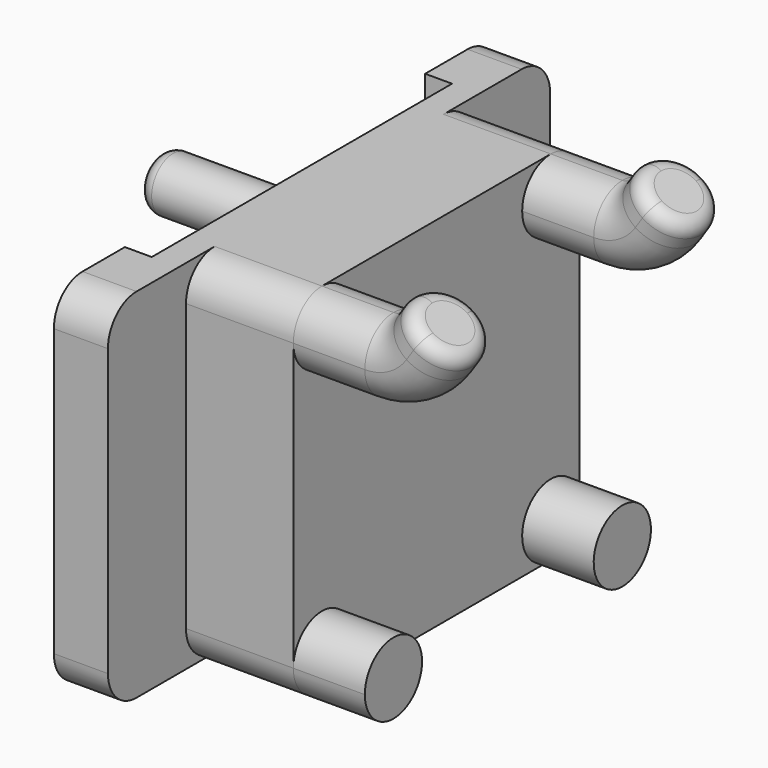
from build123d import *

# Parameters (mm, degrees)
F0_W      = 31.75
F0_H      = 31.75
F1_DEPTH  = 9.525
F7_R      = 1.27
F11_DEPTH = 6.35
F12_R     = 3.1749
F14_DEPTH = 4.8006
F15_W     = 33.3248
F15_H     = 31.75
F16_DEPTH = 2.3876
F17_R     = 2.3876
F18_DEPTH = 12.7
F19_R     = 3.175
F20_R     = 1.27


# Not quite as in the source:
# - a fillet or chamfer is up to 0.001 mm smaller than in the source, because OpenCascade refuses the exact size


with BuildPart() as f1:
    # F0 (on Right) → F1 (new body)
    with BuildSketch(Plane.YZ):
        Rectangle(F0_W, F0_H)
    extrude(amount=F1_DEPTH)

    # F6: sweep along a path in F5
    with BuildLine(Plane.XZ.offset(12.7)) as f6_path:
        Line((9.525, 9.525), (15.875, 9.525))
        ThreePointArc((15.875, 9.525), (19.4783384003, 10.4308096264), (22.225, 12.9328865162))
        Line((22.225, 12.9328865162), (23.5505334947, 14.9312034475))
    # F2 (on face) → F6 (sweep)
    with BuildSketch(Plane.YZ.offset(9.525)):
        with BuildLine():
            ThreePointArc((-15.875, 12.7), (-12.7, 9.525), (-9.525, 12.7))
            ThreePointArc((-9.525, 12.7), (-10.4549359718, 14.9450640323), (-12.7000000057, 15.875))
            ThreePointArc((-12.7000000057, 15.875), (-14.9450640323, 14.9450640282), (-15.875, 12.7))
        make_face()
    sweep(path=f6_path.line)

    # F7
    f7_edges = [f1.edges().sort_by_distance(p)[0] for p in [
        (20.9047, -15.875, 16.686251),
    ]]
    fillet(f7_edges, radius=F7_R)

    # F10: F1 across plane


with BuildPart() as f1_1:
    add(f1.part)
    add(f1.part.mirror(Plane(origin=(0, 0, 15.875), x_dir=(1, 0, 0), z_dir=(0, -1, 0))))

    # F2 (on face) → F11 (join)
    with BuildSketch(Plane.YZ.offset(9.525)):
        with BuildLine():
            ThreePointArc((-9.525, -12.7), (-12.7, -9.525), (-15.875, -12.7))
            ThreePointArc((-15.875, -12.7), (-14.9450640303, -14.9450640303), (-12.7, -15.875))
            ThreePointArc((-12.7, -15.875), (-10.4549359697, -14.9450640303), (-9.525, -12.7))
        make_face()
        with BuildLine():
            ThreePointArc((12.7, -15.875), (14.9450640303, -14.9450640303), (15.875, -12.7))
            ThreePointArc((15.875, -12.7), (10.4549359697, -10.4549359697), (12.7, -15.875))
        make_face()
    extrude(amount=F11_DEPTH)

    # F12 (radius 3.175 in the source; OpenCascade refuses exactly that, so slightly less here)
    f12_edges = [f1_1.edges().sort_by_distance(p)[0] for p in [
        (4.7625, -15.875, 15.875),
        (4.7625, -15.875, -15.875),
        (4.7625, 15.875, -15.875),
        (4.7625, 15.875, 15.875),
    ]]
    fillet(f12_edges, radius=F12_R)

    # F13 (on face) → F14 (join)
    with BuildSketch(Plane(origin=(0, 0, 0), x_dir=(0, -1, 0), z_dir=(-1, 0, 0))):
        with BuildLine():
            Line((-12.7001, 15.875), (-24.5396645936, 15.875))
            Line((-24.5396645936, 15.875), (-24.5396645936, -15.875))
            Line((-24.5396645936, -15.875), (-12.7001, -15.875))
            ThreePointArc((-12.7001, -15.875), (-14.9450933196, -14.9450933196), (-15.875, -12.7001))
            Line((-15.875, -12.7001), (-15.875, 12.7001))
            ThreePointArc((-15.875, 12.7001), (-14.9450933196, 14.9450933196), (-12.7001, 15.875))
        make_face()
        with BuildLine():
            Line((12.7001, 15.875), (-12.7001, 15.875))
            ThreePointArc((-12.7001, 15.875), (-14.9450933196, 14.9450933196), (-15.875, 12.7001))
            Line((-15.875, 12.7001), (-15.875, -12.7001))
            ThreePointArc((-15.875, -12.7001), (-14.9450933196, -14.9450933196), (-12.7001, -15.875))
            Line((-12.7001, -15.875), (12.7001, -15.875))
            ThreePointArc((12.7001, -15.875), (14.9450933196, -14.9450933196), (15.875, -12.7001))
            Line((15.875, -12.7001), (15.875, 12.7001))
            ThreePointArc((15.875, 12.7001), (14.9450933196, 14.9450933196), (12.7001, 15.875))
        make_face()
        with BuildLine():
            Line((24.5396645936, 15.875), (12.7001, 15.875))
            ThreePointArc((12.7001, 15.875), (14.9450933196, 14.9450933196), (15.875, 12.7001))
            Line((15.875, 12.7001), (15.875, -12.7001))
            ThreePointArc((15.875, -12.7001), (14.9450933196, -14.9450933196), (12.7001, -15.875))
            Line((12.7001, -15.875), (24.5396645936, -15.875))
            Line((24.5396645936, -15.875), (24.5396645936, 15.875))
        make_face()
    extrude(amount=F14_DEPTH)

    # F15 (on face) → F16 (cut)
    with BuildSketch(Plane(origin=(-4.8006, 0, 0), x_dir=(0, -1, 0), z_dir=(-1, 0, 0))):
        Rectangle(F15_W, F15_H)
    extrude(amount=-F16_DEPTH, mode=Mode.SUBTRACT)

    # F17 (on face) → F18 (join)
    with BuildSketch(Plane(origin=(-2.413, 0, 0), x_dir=(0, -1, 0), z_dir=(-1, 0, 0))):
        with Locations((0, 11.0998)):
            Circle(F17_R)
    extrude(amount=F18_DEPTH)

    # F19
    f19_edges = [f1_1.edges().sort_by_distance(p)[0] for p in [
        (-2.4003, 24.539665, 15.875),
        (-2.4003, 24.539665, -15.875),
        (-2.4003, -24.539665, -15.875),
        (-2.4003, -24.539665, 15.875),
    ]]
    fillet(f19_edges, radius=F19_R)

    # F20
    f20_edges = [f1_1.edges().sort_by_distance(p)[0] for p in [
        (-15.113, 2.3876, 11.0998),
    ]]
    fillet(f20_edges, radius=F20_R)


solid = f1_1.part
